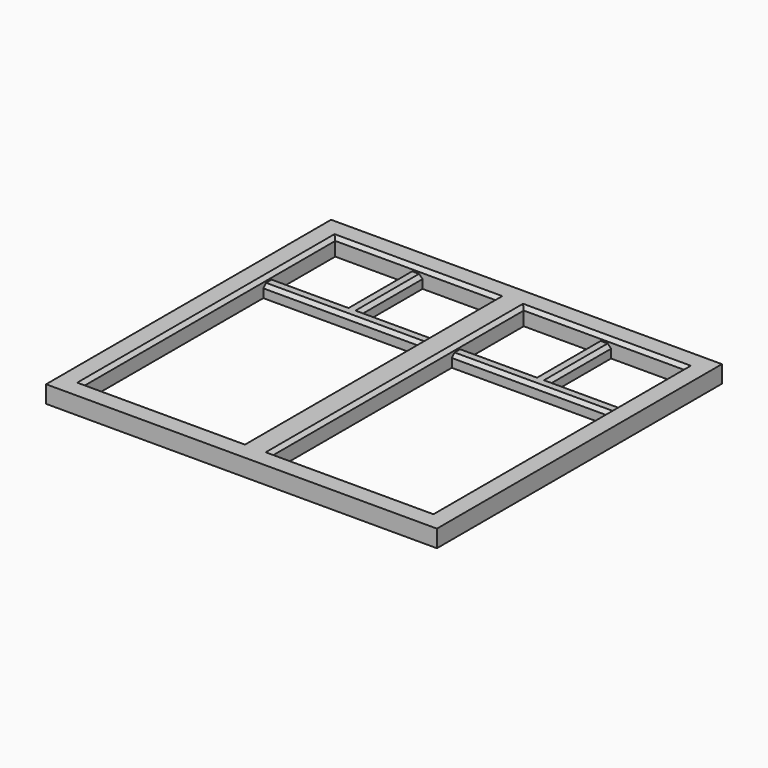
from build123d import *

# Parameters (mm, degrees)
F0_W      = 1130
F0_H      = 1030
F1_DEPTH  = 50
F2_DEPTH  = 35
F3_SIZE   = 10
F3_2_SIZE = 10
F3_3_SIZE = 10


with BuildPart() as f1:
    # F0 (on Top) → F1 (new body)
    with BuildSketch(Plane.XY):
        with Locations((285.3141621128, 160.2047318473)):
            Rectangle(F0_W, F0_H)
        Polygon((-219.6858378872, -294.7952681527), (-219.6858378872, 355.2047318473), (-219.6858378872, 395.2047318473), (-219.6858378872, 615.2047318473), (-7.1858378872, 615.2047318473), (32.8141621128, 615.2047318473), (245.3141621128, 615.2047318473), (245.3141621128, 395.2047318473), (245.3141621128, 355.2047318473), (245.3141621128, -294.7952681527), align=None, mode=Mode.SUBTRACT)
        Polygon((325.3141621128, -294.7952681527), (325.3141621128, 355.2047318473), (325.3141621128, 395.2047318473), (325.3141621128, 615.2047318473), (537.8141621128, 615.2047318473), (577.8141621128, 615.2047318473), (790.3141621128, 615.2047318473), (790.3141621128, 395.2047318473), (790.3141621128, 355.2047318473), (790.3141621128, -294.7952681527), align=None, mode=Mode.SUBTRACT)
    extrude(amount=F1_DEPTH)

    # F3
    f3_edges = [f1.edges().sort_by_distance(p)[0] for p in [
        (-219.685838, 160.204732, 50),
        (12.814162, 615.204732, 50),
        (245.314162, 160.204732, 50),
        (325.314162, 160.204732, 50),
        (557.814162, 615.204732, 50),
        (790.314162, 160.204732, 50),
        (557.814162, -294.795268, 50),
        (12.814162, -294.795268, 50),
    ]]
    chamfer(f3_edges, length=F3_SIZE)


with BuildPart() as f2:
    # F0 (on Top) → F2 (new body)
    with BuildSketch(Plane.XY):
        Polygon((-219.6858378872, 395.2047318473), (-219.6858378872, 355.2047318473), (245.3141621128, 355.2047318473), (245.3141621128, 395.2047318473), (32.8141621128, 395.2047318473), (32.8141621128, 615.2047318473), (-7.1858378872, 615.2047318473), (-7.1858378872, 395.2047318473), align=None)
    extrude(amount=F2_DEPTH)

    # F3#2
    f3_2_edges = [f2.edges().sort_by_distance(p)[0] for p in [
        (12.814162, 355.204732, 35),
        (139.064162, 395.204732, 35),
        (32.814162, 505.204732, 35),
        (-7.185838, 505.204732, 35),
        (-113.435838, 395.204732, 35),
    ]]
    chamfer(f3_2_edges, length=F3_2_SIZE)


with BuildPart() as f2b:
    # F0 (on Top) → F2, piece 2 (new body)
    with BuildSketch(Plane.XY):
        Polygon((325.3141621128, 395.2047318473), (325.3141621128, 355.2047318473), (790.3141621128, 355.2047318473), (790.3141621128, 395.2047318473), (577.8141621128, 395.2047318473), (577.8141621128, 615.2047318473), (537.8141621128, 615.2047318473), (537.8141621128, 395.2047318473), align=None)
    extrude(amount=F2_DEPTH)

    # F3#3
    f3_3_edges = [f2b.edges().sort_by_distance(p)[0] for p in [
        (557.814162, 355.204732, 35),
        (431.564162, 395.204732, 35),
        (577.814162, 505.204732, 35),
        (684.064162, 395.204732, 35),
        (537.814162, 505.204732, 35),
    ]]
    chamfer(f3_3_edges, length=F3_3_SIZE)


solid = Compound([f1.part, f2.part, f2b.part])
